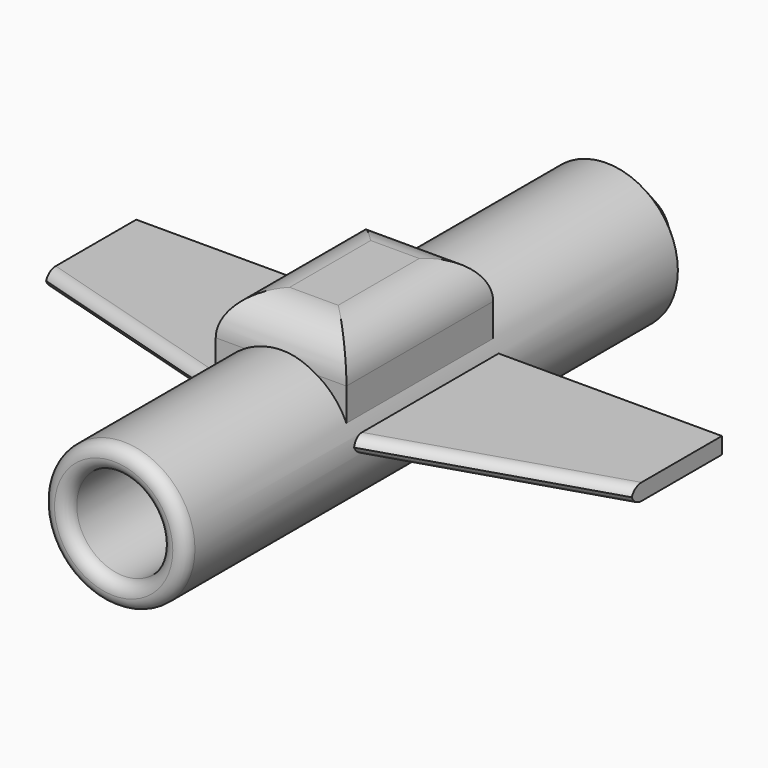
from build123d import *

# Parameters (mm, degrees)
F0_R          = 44.1944447312
F1_DEPTH      = 330.2
F2_T          = -15.24
F3_R          = 7.61999
F4_DEPTH      = 76.2
F5_SIZE       = 25.4
F6_W          = 80.8569788933
F6_H          = 113.4834885597
F7_DEPTH      = 63.5
F8_T1_DEPTH   = 240.4834885597
F8_T6_DEPTH   = 207.8569788933
F8_S7_R       = 44.1944447312
F8_T8_DEPTH   = 107
F8_T12_DEPTH  = 207.8569788933
F8_S13_R      = 44.1944447312
F8_T14_DEPTH  = 107
F10_DEPTH     = 10.16
F11_T4_DEPTH  = 181.6717263284
F11_S5_R      = 44.1944447312
F11_T6_DEPTH  = 95
F11_T10_DEPTH = 182.9126104381
F11_S11_R     = 44.1944447312
F11_T12_DEPTH = 95
F11_T16_DEPTH = 182.201088869
F11_S17_R     = 44.1944447312
F11_T18_DEPTH = 95
F11_T22_DEPTH = 180.9663017132
F11_S23_R     = 44.1944447312
F11_T24_DEPTH = 94


# Not quite as in the source:
# - a fillet or chamfer that OpenCascade refuses, or shapes differently, is made with other operations: its cross-section is extruded or revolved along the edge and cut away or added
# - a fillet or chamfer is up to 0.001 mm smaller than in the source, because OpenCascade refuses the exact size


with BuildPart() as f1:
    # F0 (on Front) → F1 (new body)
    with BuildSketch(Plane.XZ):
        Circle(F0_R)
    extrude(amount=F1_DEPTH)

    # F2
    f2_openings = [f1.faces().sort_by_distance(p)[0] for p in [
        (0, -330.2, 0),
    ]]
    offset(amount=F2_T, openings=f2_openings)

    # F3 (radius 7.62 in the source; OpenCascade refuses exactly that, so slightly less here)
    f3_edges = [f1.edges().sort_by_distance(p)[0] for p in [
        (-44.194445, -330.2, 0),
        (-28.954445, -330.2, 0),
    ]]
    fillet(f3_edges, radius=F3_R)

    # F4 (add): a face of the model
    f4_faces = [f1.faces().sort_by_distance(p)[0] for p in [
        (0, 0, 0),
    ]]
    extrude(f4_faces, amount=F4_DEPTH)

    # F5
    f5_edges = [f1.edges().sort_by_distance(p)[0] for p in [
        (-44.194445, 76.2, 0),
    ]]
    chamfer(f5_edges, length=F5_SIZE)

    # F6 (on Top) → F7 (join)
    with BuildSketch(Plane.XY):
        with Locations((0, -144.0225243568)):
            Rectangle(F6_W, F6_H)
    extrude(amount=F7_DEPTH)

    # F8: fillet of radius 25.4 on 4 edges, made by hand

    # F8_s2 → F8_t1 (cut)
    with BuildSketch(Plane.XZ.offset(23.780780077)):
        with BuildLine():
            ThreePointArc((40.4284894466, 38.1), (32.9890016888, 56.0605122421), (15.0284894466, 63.5))
            Line((15.0284894466, 63.5), (40.4284894466, 63.5))
            Line((40.4284894466, 63.5), (40.4284894466, 38.1))
        make_face()
        with BuildLine():
            ThreePointArc((-40.4284894466, 38.1), (-32.9890016888, 56.0605122421), (-15.0284894466, 63.5))
            Line((-15.0284894466, 63.5), (-40.4284894466, 63.5))
            Line((-40.4284894466, 63.5), (-40.4284894466, 38.1))
        make_face()
    extrude(amount=F8_T1_DEPTH, mode=Mode.SUBTRACT)


with BuildPart() as f8_tool4:
    # F8_s5 → F8_t6 (new body)
    with BuildSketch(Plane.YZ.offset(103.9284894466)):
        with BuildLine():
            ThreePointArc((-87.280780077, 38.1), (-94.7202678348, 56.0605122421), (-112.680780077, 63.5))
            Line((-112.680780077, 63.5), (-87.280780077, 63.5))
            Line((-87.280780077, 63.5), (-87.280780077, 38.1))
        make_face()
    extrude(amount=-F8_T6_DEPTH)

    # F8_s7 → F8_t8 (cut, symmetric)
    with BuildSketch(Plane.XZ.offset(100)):
        Circle(F8_S7_R)
    extrude(amount=F8_T8_DEPTH, both=True, mode=Mode.SUBTRACT)


with BuildPart() as f1_1:
    add(f1.part)

    # F8_t3: cut F8_tool4
    add(f8_tool4.part, mode=Mode.SUBTRACT)


with BuildPart() as f8_tool10:
    # F8_s11 → F8_t12 (new body)
    with BuildSketch(Plane.YZ.offset(-103.9284894466)):
        with BuildLine():
            ThreePointArc((-200.7642686367, 38.1), (-193.3247808788, 56.0605122421), (-175.3642686367, 63.5))
            Line((-175.3642686367, 63.5), (-200.7642686367, 63.5))
            Line((-200.7642686367, 63.5), (-200.7642686367, 38.1))
        make_face()
    extrude(amount=F8_T12_DEPTH)

    # F8_s13 → F8_t14 (cut, symmetric)
    with BuildSketch(Plane.XZ.offset(188.1)):
        Circle(F8_S13_R)
    extrude(amount=F8_T14_DEPTH, both=True, mode=Mode.SUBTRACT)


with BuildPart() as f1_2:
    add(f1_1.part)

    # F8_t9: cut F8_tool10
    add(f8_tool10.part, mode=Mode.SUBTRACT)

    # F9 (on Top) → F10 (join)
    with BuildSketch(Plane.XY):
        Polygon((181.1510026455, -156.4789265394), (181.1510026455, -86.3388031721), (-181.1510026455, -86.3388031721), (-181.1510026455, -156.4789265394), (-40.541768074, -156.4789265394), (40.4533445835, -156.4789265394), align=None)
        Polygon((40.4533445835, -200.733974576), (181.1510026455, -156.4789265394), (40.4533445835, -156.4789265394), align=None)
        Polygon((-40.541768074, -156.4789265394), (-181.1510026455, -156.4789265394), (-40.541768074, -198.22897017), align=None)
    extrude(amount=F10_DEPTH)

    # F11: fillet of radius 7.62 on 4 edges, made by hand


with BuildPart() as f11_tool2:
    # F11_s3 → F11_t4 (new body)
    with BuildSketch(Plane(origin=(-35.0743442089, -11.0322858902, 0), x_dir=(0, 0, 1), z_dir=(0.9539242957, 0.3000473932, 0))):
        with BuildLine():
            ThreePointArc((0, 196.0029358997), (2.2318463274, 201.3910895724), (7.62, 203.6229358997))
            Line((7.62, 203.6229358997), (0, 203.6229358997))
            Line((0, 203.6229358997), (0, 196.0029358997))
        make_face()
    extrude(amount=F11_T4_DEPTH)

    # F11_s5 → F11_t6 (cut, symmetric)
    with BuildSketch(Plane.XZ.offset(174.4)):
        Circle(F11_S5_R)
    extrude(amount=F11_T6_DEPTH, both=True, mode=Mode.SUBTRACT)


with BuildPart() as f1_3:
    add(f1_2.part)

    # F11_t1: cut F11_tool2
    add(f11_tool2.part, mode=Mode.SUBTRACT)


with BuildPart() as f11_tool8:
    # F11_s9 → F11_t10 (new body)
    with BuildSketch(Plane(origin=(-36.2580537092, -11.4046099325, 0), x_dir=(0, 0, 1), z_dir=(0.9539242957, 0.3000473932, 0))):
        with BuildLine():
            ThreePointArc((2.54, 203.6229358997), (7.9281536726, 201.3910895724), (10.16, 196.0029358997))
            Line((10.16, 196.0029358997), (10.16, 203.6229358997))
            Line((10.16, 203.6229358997), (2.54, 203.6229358997))
        make_face()
    extrude(amount=F11_T10_DEPTH)

    # F11_s11 → F11_t12 (cut, symmetric)
    with BuildSketch(Plane.XZ.offset(174.6)):
        Circle(F11_S11_R)
    extrude(amount=F11_T12_DEPTH, both=True, mode=Mode.SUBTRACT)


with BuildPart() as f1_4:
    add(f1_3.part)

    # F11_t7: cut F11_tool8
    add(f11_tool8.part, mode=Mode.SUBTRACT)


with BuildPart() as f11_tool14:
    # F11_s15 → F11_t16 (new body)
    with BuildSketch(Plane(origin=(-142.0383828725, 42.1743898985, 0), x_dir=(0, 0, 1), z_dir=(0.9586344454, -0.2846401237, 0))):
        with BuildLine():
            ThreePointArc((10.16, 193.9489327682), (7.9281536726, 199.3370864408), (2.54, 201.5689327682))
            Line((2.54, 201.5689327682), (10.16, 201.5689327682))
            Line((10.16, 201.5689327682), (10.16, 193.9489327682))
        make_face()
    extrude(amount=F11_T16_DEPTH)

    # F11_s17 → F11_t18 (cut, symmetric)
    with BuildSketch(Plane.XZ.offset(173.3)):
        Circle(F11_S17_R)
    extrude(amount=F11_T18_DEPTH, both=True, mode=Mode.SUBTRACT)


with BuildPart() as f1_5:
    add(f1_4.part)

    # F11_t13: cut F11_tool14
    add(f11_tool14.part, mode=Mode.SUBTRACT)


with BuildPart() as f11_tool20:
    # F11_s21 → F11_t22 (new body)
    with BuildSketch(Plane(origin=(-142.0383828725, 42.1743898985, 0), x_dir=(0, 0, 1), z_dir=(0.9586344454, -0.2846401237, 0))):
        with BuildLine():
            ThreePointArc((7.62, 201.5689327682), (2.2318463274, 199.3370864408), (0, 193.9489327682))
            Line((0, 193.9489327682), (0, 201.5689327682))
            Line((0, 201.5689327682), (7.62, 201.5689327682))
        make_face()
    extrude(amount=F11_T22_DEPTH)

    # F11_s23 → F11_t24 (cut, symmetric)
    with BuildSketch(Plane.XZ.offset(173.2)):
        Circle(F11_S23_R)
    extrude(amount=F11_T24_DEPTH, both=True, mode=Mode.SUBTRACT)


with BuildPart() as f1_6:
    add(f1_5.part)

    # F11_t19: cut F11_tool20
    add(f11_tool20.part, mode=Mode.SUBTRACT)


solid = f1_6.part
